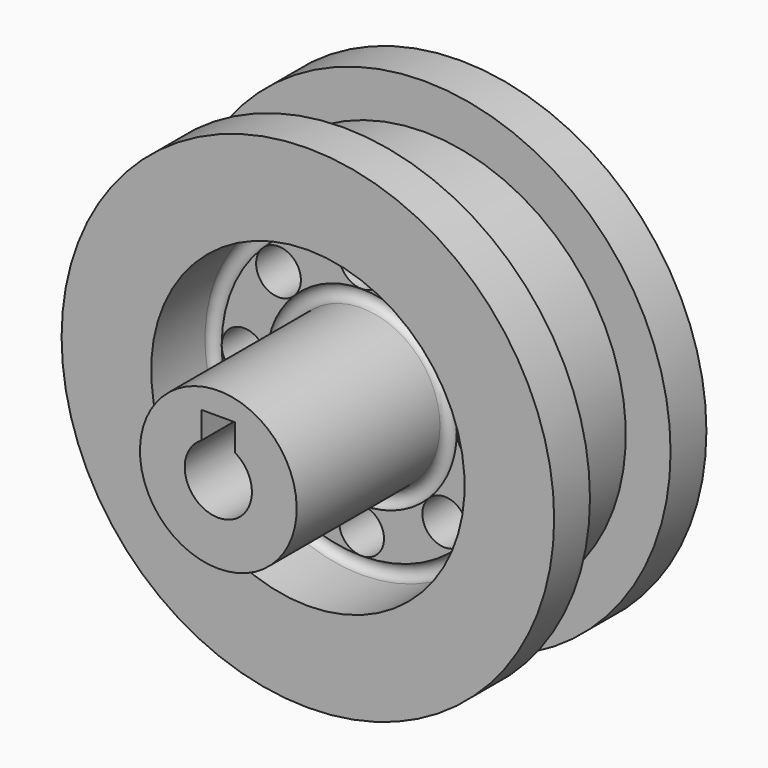
from build123d import *

# Parameters (mm, degrees)
F2_W     = 3
F2_H     = 2.4007145502
F4_DEPTH = 23
F3_R     = 2
F5_DEPTH = 4
F7_R     = 0.75
F9_R     = 0.75


with BuildPart() as f1:
    # F0 (on Right) → F1 (revolve)
    with BuildSketch(Plane.YZ):
        Polygon((23, -3), (0, -3), (0, -7), (16, -7), (16, -14), (10, -14), (10, -22), (14, -22), (14, -18), (23, -18), (23, -22), (27, -22), (27, -14), (20, -14), (20, -7), (23, -7), align=None)
    revolve(axis=Axis((0, 11.4535925208, 0), (0, 1, 0)))

    # F2 (on Front) → F4 (cut, through all)
    with BuildSketch(Plane.XZ):
        with Locations((0, 3.7996427249)):
            Rectangle(F2_W, F2_H)
    extrude(amount=-F4_DEPTH, mode=Mode.SUBTRACT)

    # F3 (on face) → F5 (cut, through all)
    with BuildSketch(Plane.XZ.offset(-16)):
        with Locations((0, 10.5)):
            Circle(F3_R)
        with Locations((7.4246212025, 7.4246212025)):
            Circle(F3_R)
        with Locations((10.5, 0)):
            Circle(F3_R)
        with Locations((7.4246212025, -7.4246212025)):
            Circle(F3_R)
        with Locations((0, -10.5)):
            Circle(F3_R)
        with Locations((-7.4246212025, -7.4246212025)):
            Circle(F3_R)
        with Locations((-10.5, 0)):
            Circle(F3_R)
        with Locations((-7.4246212025, 7.4246212025)):
            Circle(F3_R)
    extrude(amount=-F5_DEPTH, mode=Mode.SUBTRACT)

    # F8: sweep along a path in F6
    with BuildLine(Plane.XZ.offset(-16)) as f8_path:
        CenterArc((0, 0), 13.25, 0, 360)
    # F7 (on Top) → F8 (sweep, cut)
    with BuildSketch(Plane.XY):
        with Locations((13.25, 16)):
            Circle(F7_R)
    sweep(path=f8_path.line, mode=Mode.SUBTRACT)

    # F11: sweep along a path in F10
    with BuildLine(Plane.XZ.offset(-16)) as f11_path:
        CenterArc((0, 0), 7.75, 0, 360)
    # F9 (on Top) → F11 (sweep, cut)
    with BuildSketch(Plane.XY):
        with Locations((7.75, 16)):
            Circle(F9_R)
    sweep(path=f11_path.line, mode=Mode.SUBTRACT)


solid = f1.part
